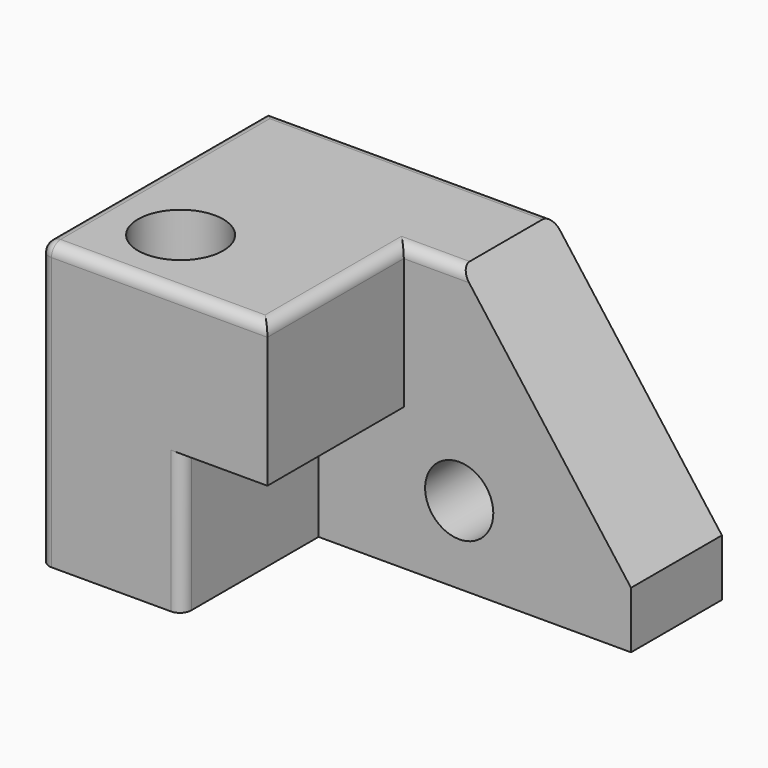
from build123d import *

# Parameters (mm, degrees)
F0_W        = 203.2
F0_H        = 127
F1_DEPTH    = 127
F3_DEPTH    = 76.2
F4_SIZE2    = 101.6
F4_SIZE     = 76.2
F5_R        = 5.08
F6_T1_DEPTH = 76.2
F6_T3_DEPTH = 134.62
F6_S7_W     = 5.08
F6_S7_H     = 5.08
F6_T8_DEPTH = 5.08
F7_R        = 15.24
F8_DEPTH    = 50.8
F9_R        = 19.05
F10_DEPTH   = 127


# Not quite as in the source:
# - a fillet or chamfer that OpenCascade refuses, or shapes differently, is made with other operations: its cross-section is extruded or revolved along the edge and cut away or added


with BuildPart() as f1:
    # F0 (on Front) → F1 (new body)
    with BuildSketch(Plane.XZ):
        with Locations((12.863317194, -0.4497872638)):
            Rectangle(F0_W, F0_H)
    extrude(amount=F1_DEPTH)

    # F2 (on face) → F3 (cut)
    with BuildSketch(Plane.XZ.offset(127)):
        Polygon((114.463317194, 63.0502127362), (12.863317194, 63.0502127362), (12.863317194, -0.4497872638), (-25.236682806, -0.4497872638), (-25.236682806, -63.9497872638), (114.463317194, -63.9497872638), align=None)
    extrude(amount=-F3_DEPTH, mode=Mode.SUBTRACT)

    # F4
    f4_edges = [f1.edges().sort_by_distance(p)[0] for p in [
        (114.463317, -25.4, 63.050213),
    ]]
    f4_side = f1.faces().sort_by_distance((-8.908111, -52.614286, 63.050213))[0]
    chamfer(f4_edges, length=F4_SIZE, length2=F4_SIZE2, reference=f4_side)

    # F5
    f5_edges = [f1.edges().sort_by_distance(p)[0] for p in [
        (-37.936683, -127, 63.050213),
        (-88.736683, -63.5, 63.050213),
        (12.863317, -88.9, 63.050213),
        (25.563317, -50.8, 63.050213),
        (-25.236683, 0, 63.050213),
    ]]
    fillet(f5_edges, radius=F5_R)

    # F6: fillet of radius 5.08 on 2 edges, made by hand

    # F6_s2 → F6_t1 (cut)
    with BuildSketch(Plane.XY.offset(-76.6497872638)):
        with BuildLine():
            ThreePointArc((-30.316682806, -127), (-26.7245803576, -125.5121024484), (-25.236682806, -121.92))
            Line((-25.236682806, -121.92), (-25.236682806, -127))
            Line((-25.236682806, -127), (-30.316682806, -127))
        make_face()
    extrude(amount=F6_T1_DEPTH, mode=Mode.SUBTRACT)

    # F6_s4 → F6_t3 (cut)
    with BuildSketch(Plane.XY.offset(-76.6497872638)):
        with BuildLine():
            ThreePointArc((-88.736682806, -121.92), (-87.2487852545, -125.5121024484), (-83.656682806, -127))
            Line((-83.656682806, -127), (-88.736682806, -127))
            Line((-88.736682806, -127), (-88.736682806, -121.92))
        make_face()
    extrude(amount=F6_T3_DEPTH, mode=Mode.SUBTRACT)


with BuildPart() as f6_tool6:
    # F6_s7 → F6_t8 (new body)
    with BuildSketch(Plane.YZ.offset(-83.656682806)):
        with Locations((-124.46, 60.5102127362)):
            Rectangle(F6_S7_W, F6_S7_H)
    extrude(amount=-F6_T8_DEPTH)

    # F6_s9 → F6_t10 (revolve, cut)
    with BuildSketch(Plane(origin=(-83.656682806, -121.92, 57.9702127362), x_dir=(0, 0.7071067812, -0.7071067812), z_dir=(0, 0.7071067812, 0.7071067812))):
        with BuildLine():
            ThreePointArc((0, -5.08), (5.08, 0), (0, 5.08))
            Line((0, 5.08), (0, -5.08))
        make_face()
    revolve(axis=Axis((-83.656682806, -121.92, 57.9702127362), (-1, 0, 0)), mode=Mode.SUBTRACT)


with BuildPart() as f1_1:
    add(f1.part)

    # F6_t5: cut F6_tool6
    add(f6_tool6.part, mode=Mode.SUBTRACT)

    # F7 (on face) → F8 (cut, through all)
    with BuildSketch(Plane.XZ.offset(50.8)):
        with Locations((37.6529693604, -29.2071215808)):
            Circle(F7_R)
    extrude(amount=-F8_DEPTH, mode=Mode.SUBTRACT)

    # F9 (on face) → F10 (cut, through all)
    with BuildSketch(Plane.XY.offset(63.0502127362)):
        with Locations((-53.0607067049, -93.1101441383)):
            Circle(F9_R)
    extrude(amount=-F10_DEPTH, mode=Mode.SUBTRACT)


solid = f1_1.part
